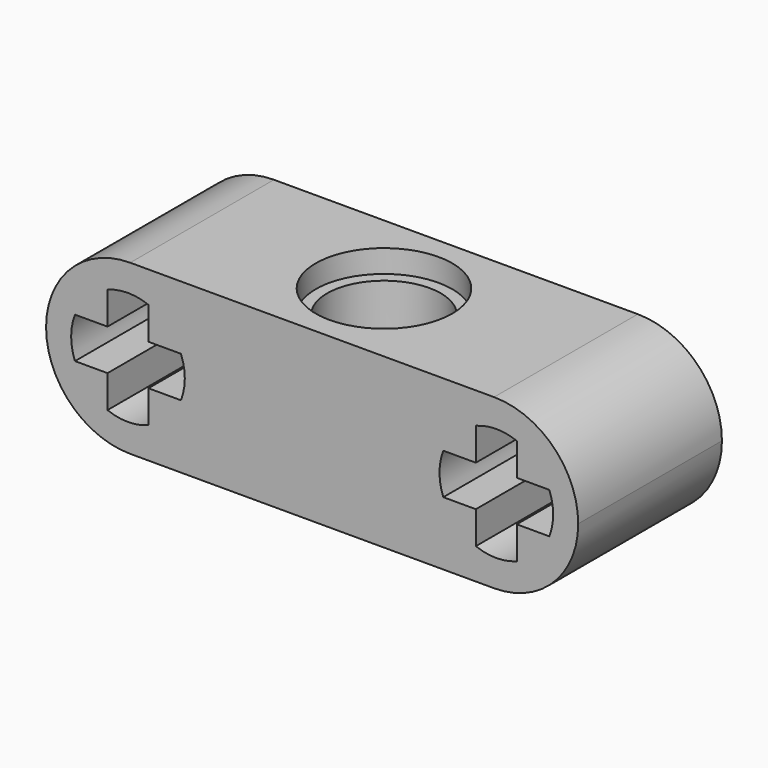
from build123d import *

# Parameters (mm, degrees)
F0_W     = 23.4
F0_H     = 7.4
F1_DEPTH = 3.95
F2_R     = 3.69999
F3_R     = 2.499
F4_DEPTH = 25
F3_R_2   = 3
F5_DEPTH = 1
F6_R     = 3
F6_R_2   = 2.499
F7_DEPTH = 1


# Not quite as in the source:
# - a fillet or chamfer is up to 0.001 mm smaller than in the source, because OpenCascade refuses the exact size


with BuildPart() as f1:
    # F0 (on Front) → F1 (new body, symmetric)
    with BuildSketch(Plane.XZ):
        Rectangle(F0_W, F0_H)
        with BuildLine():
            ThreePointArc((-7.199, -2.3313088598), (-8.099, -2.499), (-8.999, -2.3313088598))
            Line((-8.999, -2.3313088598), (-8.999, -0.9))
            Line((-8.999, -0.9), (-10.4303088598, -0.9))
            ThreePointArc((-10.4303088598, -0.9), (-10.598, 0), (-10.4303088598, 0.9))
            Line((-10.4303088598, 0.9), (-8.999, 0.9))
            Line((-8.999, 0.9), (-8.999, 2.3313088598))
            ThreePointArc((-8.999, 2.3313088598), (-8.099, 2.499), (-7.199, 2.3313088598))
            Line((-7.199, 2.3313088598), (-7.199, 0.9))
            Line((-7.199, 0.9), (-5.7676911402, 0.9))
            ThreePointArc((-5.7676911402, 0.9), (-5.6, 0), (-5.7676911402, -0.9))
            Line((-5.7676911402, -0.9), (-7.199, -0.9))
            Line((-7.199, -0.9), (-7.199, -2.3313088598))
        make_face(mode=Mode.SUBTRACT)
        with BuildLine():
            Line((7.199, 0.9), (7.199, 2.3313088598))
            ThreePointArc((7.199, 2.3313088598), (8.099, 2.499), (8.999, 2.3313088598))
            Line((8.999, 2.3313088598), (8.999, 0.9))
            Line((8.999, 0.9), (10.4303088598, 0.9))
            ThreePointArc((10.4303088598, 0.9), (10.598, 0), (10.4303088598, -0.9))
            Line((10.4303088598, -0.9), (8.999, -0.9))
            Line((8.999, -0.9), (8.999, -2.3313088598))
            ThreePointArc((8.999, -2.3313088598), (8.099, -2.499), (7.199, -2.3313088598))
            Line((7.199, -2.3313088598), (7.199, -0.9))
            Line((7.199, -0.9), (5.7676911402, -0.9))
            ThreePointArc((5.7676911402, -0.9), (5.6, 0), (5.7676911402, 0.9))
            Line((5.7676911402, 0.9), (7.199, 0.9))
        make_face(mode=Mode.SUBTRACT)
    extrude(amount=F1_DEPTH, both=True)

    # F2 (radius 3.7 in the source; OpenCascade refuses exactly that, so slightly less here)
    f2_edges = [f1.edges().sort_by_distance(p)[0] for p in [
        (-11.7, 0, -3.7),
        (-11.7, 0, 3.7),
        (11.7, 0, 3.7),
        (11.7, 0, -3.7),
    ]]
    fillet(f2_edges, radius=F2_R)

    # F3 (on face) → F4 (cut)
    with BuildSketch(Plane.XY.offset(3.7)):
        Circle(F3_R)
    extrude(amount=-F4_DEPTH, mode=Mode.SUBTRACT)

    # F3 (on face) → F5 (cut)
    with BuildSketch(Plane.XY.offset(3.7)):
        Circle(F3_R_2)
        Circle(F3_R, mode=Mode.SUBTRACT)
    extrude(amount=-F5_DEPTH, mode=Mode.SUBTRACT)

    # F6 (on face) → F7 (cut)
    with BuildSketch(Plane(origin=(0, 0, -3.7), x_dir=(1, 0, 0), z_dir=(0, 0, -1))):
        Circle(F6_R)
        Circle(F6_R_2, mode=Mode.SUBTRACT)
    extrude(amount=-F7_DEPTH, mode=Mode.SUBTRACT)


solid = f1.part
